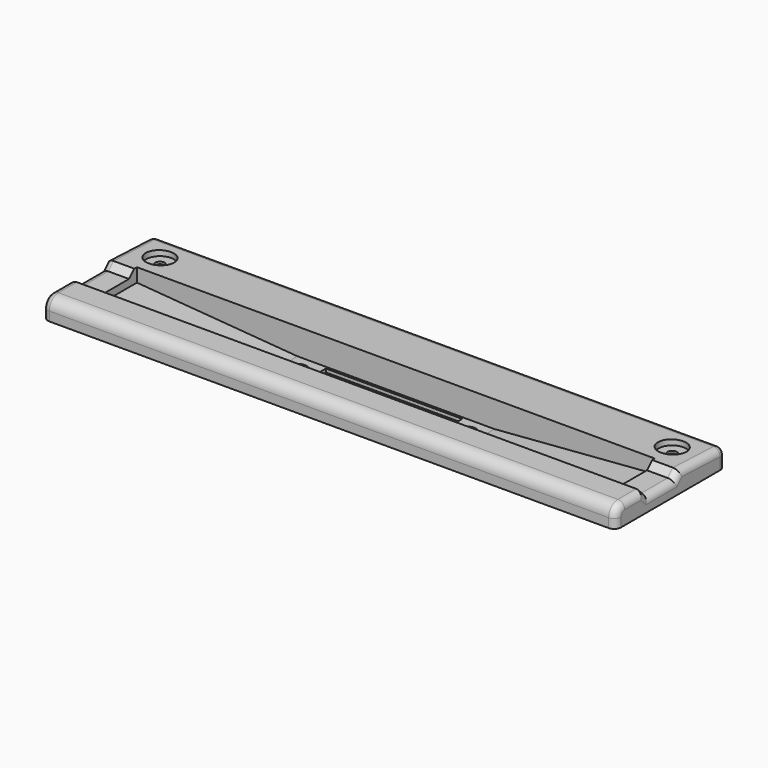
from build123d import *

# Parameters (mm, degrees)
F0_W         = 250
F0_H         = 60
F1_DEPTH     = 9
F2_W         = 86
F2_H         = 4
F3_DEPTH     = 16
F4_DEPTH     = 7.9
F5_W         = 59.5
F5_H         = 14.5
F6_DEPTH     = 13.001
F7_R         = 1.7543464605
F8_DEPTH     = 13.001
F9_W         = 246
F9_H         = 20.1
F9_H_2       = 12
F10_DEPTH    = 7
F11_R        = 1.9
F12_DEPTH    = 2.001
F14_R        = 7
F15_DEPTH    = 2
F13_R        = 6
F16_DEPTH    = 3
F17_R        = 2
F18_DEPTH    = 25
F19_W        = 86
F19_H        = 21
F20_DEPTH    = 11.5
F22_DEPTH    = 21
F24_DEPTH    = 250.001
F25_R        = 3
F26_T1_DEPTH = 250
F26_T4_ANGLE = 90
F26_T6_ANGLE = 90
F27_R        = 4
F28_DEPTH    = 1


# Not quite as in the source:
# - a fillet or chamfer that OpenCascade refuses, or shapes differently, is made with other operations: its cross-section is extruded or revolved along the edge and cut away or added


with BuildPart() as f1:
    # F0 (on Top) → F1 (new body)
    with BuildSketch(Plane.XY):
        Rectangle(F0_W, F0_H)
    extrude(amount=F1_DEPTH)

    # F2 (on Front) → F3 (join)
    with BuildSketch(Plane.XZ):
        Polygon((-43, 0), (-125, 0), (-43, -4), align=None)
        with Locations((0, -2)):
            Rectangle(F2_W, F2_H)
        Polygon((125, 0), (43, 0), (43, -4), align=None)
    extrude(amount=F3_DEPTH)

    # F2 (on Front) → F4 (join)
    with BuildSketch(Plane.XZ):
        Polygon((-43, 0), (-125, 0), (-43, -4), align=None)
        with Locations((0, -2)):
            Rectangle(F2_W, F2_H)
        Polygon((125, 0), (43, 0), (43, -4), align=None)
    extrude(amount=-F4_DEPTH)

    # F5 (on face) → F6 (cut, through all)
    with BuildSketch(Plane.XY.offset(9)):
        with Locations((0, -1.75)):
            Rectangle(F5_W, F5_H)
    extrude(amount=-F6_DEPTH, mode=Mode.SUBTRACT)

    # F7 (on face) → F8 (cut, through all)
    with BuildSketch(Plane(origin=(0, 0, -4), x_dir=(1, 0, 0), z_dir=(0, 0, -1))):
        with Locations((-37, 1)):
            Circle(F7_R)
        with Locations((37, 1)):
            Circle(F7_R)
    extrude(amount=-F8_DEPTH, mode=Mode.SUBTRACT)

    # F9 (on face) → F10 (cut)
    with BuildSketch(Plane(origin=(0, 0, 0), x_dir=(1, 0, 0), z_dir=(0, 0, -1))):
        with Locations((0, -17.95)):
            Rectangle(F9_W, F9_H)
        with Locations((0, 22)):
            Rectangle(F9_W, F9_H_2)
    extrude(amount=-F10_DEPTH, mode=Mode.SUBTRACT)

    # F11 (on face) → F12 (cut, through all)
    with BuildSketch(Plane(origin=(0, 0, 7), x_dir=(1, 0, 0), z_dir=(0, 0, -1))):
        with Locations((-111.75, -17.5)):
            Circle(F11_R)
        with Locations((111.75, -17.5)):
            Circle(F11_R)
    extrude(amount=-F12_DEPTH, mode=Mode.SUBTRACT)

    # F14 (on face) → F15 (join)
    with BuildSketch(Plane(origin=(0, 0, 7), x_dir=(1, 0, 0), z_dir=(0, 0, -1))):
        with Locations((-111.75, -17.5)):
            Circle(F14_R)
        with Locations((111.75, -17.5)):
            Circle(F14_R)
    extrude(amount=F15_DEPTH)

    # F13 (on face) → F16 (cut)
    with BuildSketch(Plane.XY.offset(9)):
        with Locations((-111.75, 17.5)):
            Circle(F13_R)
        with Locations((111.75, 17.5)):
            Circle(F13_R)
    extrude(amount=-F16_DEPTH, mode=Mode.SUBTRACT)

    # F17 (on face) → F18 (cut)
    with BuildSketch(Plane.XY.offset(6)):
        with Locations((111.75, 17.5)):
            Circle(F17_R)
        with Locations((-111.75, 17.5)):
            Circle(F17_R)
    extrude(amount=-F18_DEPTH, mode=Mode.SUBTRACT)

    # F19 (on face) → F20 (cut)
    with BuildSketch(Plane.XY.offset(9)):
        with Locations((0, -4)):
            Rectangle(F19_W, F19_H)
    extrude(amount=-F20_DEPTH, mode=Mode.SUBTRACT)

    # F21 (on face) → F22 (cut)
    with BuildSketch(Plane(origin=(0, -14.5, 0), x_dir=(-1, 0, 0), z_dir=(0, 1, 0))):
        Polygon((113, 9), (43, 9), (43, -2.5), (113, 3), align=None)
        Polygon((-43, -2.5), (-43, 9), (-113, 9), (-113, 3), align=None)
    extrude(amount=F22_DEPTH, mode=Mode.SUBTRACT)

    # F23 (on face) → F24 (cut, through all)
    with BuildSketch(Plane.YZ.offset(125)):
        Polygon((2.1715728753, 6.1715728753), (5, 9), (-15, 9), (-12.1715728753, 6.1715728753), align=None)
        Polygon((5, 9), (30, 8), (30, 9), align=None)
    extrude(amount=-F24_DEPTH, mode=Mode.SUBTRACT)

    # F25
    f25_edges = [f1.edges().sort_by_distance(p)[0] for p in [
        (125, -22.5, 9),
        (0, 30, 8),
        (-125, -22.5, 9),
        (125, -13.585786, 7.585786),
        (125, -5, 6.171573),
        (125, 3.585786, 7.585786),
        (-125, 3.585786, 7.585786),
        (-125, -5, 6.171573),
        (-125, -13.585786, 7.585786),
        (-125, 30, 4),
        (-125, -30, 4.5),
        (125, -30, 4.5),
        (125, 30, 4),
        (125, 17.5, 8.5),
        (-125, 17.5, 8.5),
    ]]
    fillet(f25_edges, radius=F25_R)

    # F26: fillet of radius 5 on 1 edges, made by hand

    # F26_s2 → F26_t1 (cut)
    with BuildSketch(Plane.YZ.offset(-125)):
        with BuildLine():
            ThreePointArc((-30, 4), (-28.5355339059, 7.5355339059), (-25, 9))
            Line((-25, 9), (-30, 9))
            Line((-30, 9), (-30, 4))
        make_face()
    extrude(amount=F26_T1_DEPTH, mode=Mode.SUBTRACT)

    # F26_s3 → F26_t4 (revolve, cut)
    with BuildSketch(Plane.XY.offset(4)):
        with BuildLine():
            ThreePointArc((-125, -27), (-124.1213203436, -29.1213203436), (-122, -30))
            Line((-122, -30), (-125, -30))
            Line((-125, -30), (-125, -27))
        make_face()
    revolve(axis=Axis((-125, -25, 4), (-1, 0, 0)), revolution_arc=F26_T4_ANGLE, mode=Mode.SUBTRACT)

    # F26_s5 → F26_t6 (revolve, cut)
    with BuildSketch(Plane.XZ.offset(25)):
        with BuildLine():
            ThreePointArc((125, 6), (124.1213203436, 8.1213203436), (122, 9))
            Line((122, 9), (125, 9))
            Line((125, 9), (125, 6))
        make_face()
    revolve(axis=Axis((125, -25, 4), (1, 0, 0)), revolution_arc=F26_T6_ANGLE, mode=Mode.SUBTRACT)

    # F27 (on face) → F28 (cut)
    with BuildSketch(Plane.XY.offset(-2.5)):
        with Locations((37, -1)):
            Circle(F27_R)
        with Locations((-37, -1)):
            Circle(F27_R)
    extrude(amount=-F28_DEPTH, mode=Mode.SUBTRACT)


solid = f1.part
